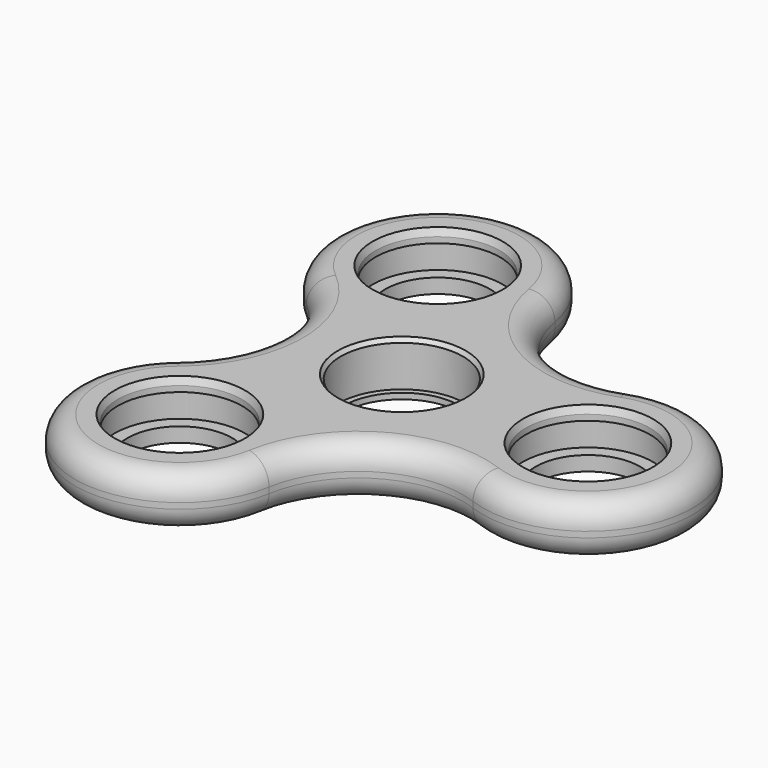
from build123d import *

# Parameters (mm, degrees)
F1_DEPTH        = 9
F5_COPIES_COUNT = 3
F6_R            = 4


# Not quite as in the source:
# - a pattern or mirror of a feature is missing from the dataset's text; its kind, count and spacing are read off the source's solid


with BuildPart() as f1:
    # F0 (on Top) → F1 (new body)
    with BuildSketch(Plane.XY):
        with BuildLine():
            ThreePointArc((1.7445626465, -30.7344840619), (10.4891252931, -18.1676979346), (25.7445626465, -16.8780776013))
            ThreePointArc((25.7445626465, -16.8780776013), (50, 0), (25.7445626465, 16.8780776013))
            ThreePointArc((25.7445626465, 16.8780776013), (10.4891252931, 18.1676979346), (1.7445626465, 30.7344840619))
            ThreePointArc((1.7445626465, 30.7344840619), (-25, 43.3012701892), (-27.4891252931, 13.8564064606))
            ThreePointArc((-27.4891252931, 13.8564064606), (-20.9782505862, 0), (-27.4891252931, -13.8564064606))
            ThreePointArc((-27.4891252931, -13.8564064606), (-25, -43.3012701892), (1.7445626465, -30.7344840619))
        make_face()
    extrude(amount=F1_DEPTH)

    # F2 (on Right) → F3 (revolve, cut)
    with BuildSketch(Plane.YZ):
        Polygon((0, 9), (0, 0), (10, 0), (10, 1), (11, 1), (11, 8.3), (10.5, 8.3), (11, 9), align=None)
    revolve(axis=Axis((0, 0, 3.7751235068), (0, 0, -1)), mode=Mode.SUBTRACT)

    # F4 (on Front) → F5 (revolve, cut)
    with BuildSketch(Plane.XZ):
        Polygon((23, 0), (32, 0), (32, 9), (20.8, 9), (21.3, 7.8), (21.3, 6.8), (20.8, 6.8), (20.8, 2.5), (23, 2.5), align=None)
    f5 = revolve(axis=Axis((32, 0, 6.29213918), (0, 0, -1)), mode=Mode.SUBTRACT)

    # F5_copies: F5 ×3 about axis
    f5_copies_axis = Axis((0, 0, 0), (0, 0, 1))
    for i in range(1, F5_COPIES_COUNT):
        add(f5.rotate(f5_copies_axis, i * 360 / F5_COPIES_COUNT), mode=Mode.SUBTRACT)

    # F6
    f6_edges = [f1.edges().sort_by_distance(p)[0] for p in [
        (10.489125, 18.167698, 9),
        (10.489125, 18.167698, 0),
        (10.489125, -18.167698, 0),
        (10.489125, -18.167698, 9),
        (-25, -43.30127, 0),
        (-25, -43.30127, 9),
        (50, 0, 0),
        (50, 0, 9),
        (-20.978251, 0, 0),
        (-25, 43.30127, 0),
        (-20.978251, 0, 9),
        (-25, 43.30127, 9),
    ]]
    fillet(f6_edges, radius=F6_R)


solid = f1.part
